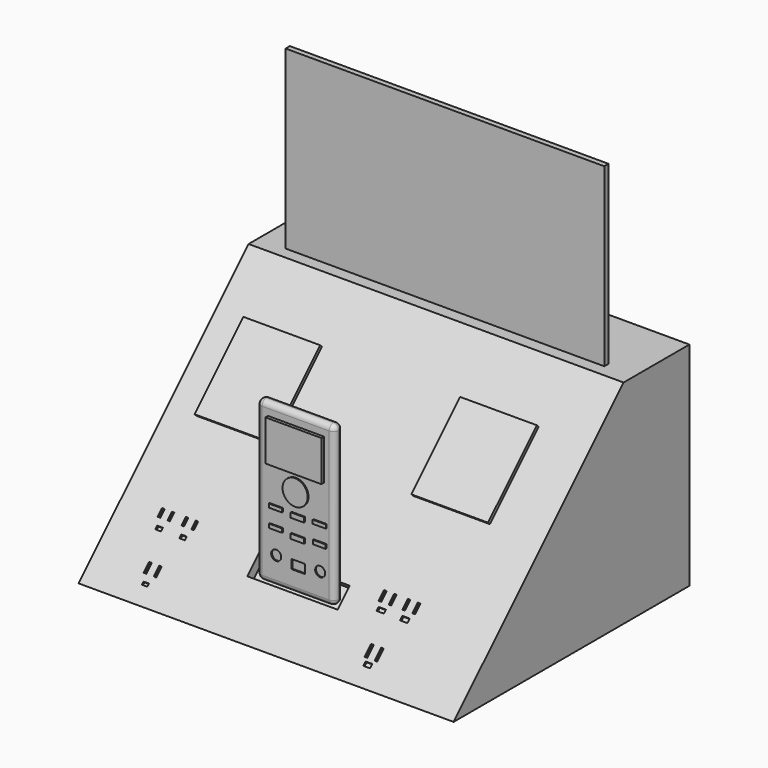
from build123d import *

# Parameters (mm, degrees)
F0_W        = 89.6722897887
F0_H        = 83.1693373621
F1_DEPTH    = 50.8
F2_T1_DEPTH = 416.2760292604
F3_W        = 76.2
F3_H        = 43.1307795863
F3_W_2      = 71.1710825562
F3_H_2      = 38.9251615852
F4_DEPTH    = 1.27
F6_W        = 18.5573295755
F6_H        = 38.1
F7_DEPTH    = 2.54
F8_R        = 1.26999
F9_W        = 21.59
F9_H        = 5.08
F10_DEPTH   = 2.286
F12_W       = 13.3995525539
F12_H       = 9.7150541842
F13_DEPTH   = 0.762
F14_R       = 3.0038864934
F14_W       = 3.1496
F14_H       = 0.8712593356
F14_W_2     = 3.1582112424
F14_H_2     = 1.159792766
F14_H_3     = 0.9281598032
F14_H_4     = 1.1401046067
F14_W_3     = 3.0329849105
F15_DEPTH   = 0.254
F14_R_2     = 1.1970137193
F14_R_3     = 1.1904625541
F14_W_4     = 3.1905571232
F14_H_5     = 2.1484075114
F16_DEPTH   = 0.254
F17_W       = 18.3596722782
F17_H       = 20.6194743514
F17_W_2     = 18.347190693
F18_DEPTH   = 0.762
F19_W       = 0.6338953972
F19_H       = 1.8462874286
F19_W_2     = 1.36038661
F19_H_2     = 0.8056527004
F19_W_3     = 0.5638897419
F19_W_4     = 0.635
F19_W_5     = 1.312000677
F19_W_6     = 0.6341952831
F19_H_3     = 2.3153796792
F19_W_7     = 1.3574287295
F19_H_4     = 0.6835795939
F19_W_8     = 1.7638131976
F19_H_5     = 0.8543668082
F19_W_9     = 1.7465222627
F19_H_6     = 0.9718833026
F19_W_10    = 1.6376990825
F19_H_7     = 0.9474921972
F19_H_8     = 2.7640033513
F19_H_9     = 2.2806219058
F20_DEPTH   = 0.508


# Not quite as in the source:
# - a fillet or chamfer that OpenCascade refuses, or shapes differently, is made with other operations: its cross-section is extruded or revolved along the edge and cut away or added
# - a fillet or chamfer is up to 0.001 mm smaller than in the source, because OpenCascade refuses the exact size
# - a feature names something its author has since deleted; it is built from what else it names


with BuildPart() as f1:
    # F0 (on Top) → F1 (new body)
    with BuildSketch(Plane.XY):
        with Locations((-0.0743344426, 4.1711423546)):
            Rectangle(F0_W, F0_H)
    extrude(amount=F1_DEPTH)

    # F2: chamfer of 63.5 on 1 edges, made by hand

    # F2_s2 → F2_t1 (cut)
    with BuildSketch(Plane.YZ.offset(-208.2123490728)):
        Polygon((-37.4135263264, -12.7), (26.0864736736, 50.8), (-37.4135263264, 50.8), align=None)
    extrude(amount=F2_T1_DEPTH, mode=Mode.SUBTRACT)

    # F9 (on face) → F10 (cut)
    with BuildSketch(Plane(origin=(0, -12.3567631632, 12.3567631632), x_dir=(1, 0, 0), z_dir=(0, -0.7071067812, 0.7071067812))):
        with Locations((-0.7835186426, -2.54)):
            Rectangle(F9_W, F9_H)
    extrude(amount=-F10_DEPTH, mode=Mode.SUBTRACT)

    # F17 (on face) → F18 (join)
    with BuildSketch(Plane(origin=(0, -12.3567631632, 12.3567631632), x_dir=(1, 0, 0), z_dir=(0, -0.7071067812, 0.7071067812))):
        with Locations((-28.8934614509, 30.5461250246)):
            Rectangle(F17_W, F17_H)
        with Locations((22.915023379, 30.5461250246)):
            Rectangle(F17_W_2, F17_H)
    extrude(amount=F18_DEPTH)

    # F19 (on face) → F20 (cut)
    with BuildSketch(Plane(origin=(0, -12.3567631632, 12.3567631632), x_dir=(1, 0, 0), z_dir=(0, -0.7071067812, 0.7071067812))):
        with Locations((-35.3719479251, 0.5594579125)):
            Rectangle(F19_W, F19_H)
        with Locations((-34.2016369104, -2.3646245245)):
            Rectangle(F19_W_2, F19_H_2)
        with Locations((-33.0321675944, 0.5594579125)):
            Rectangle(F19_W_3, F19_H)
        with Locations((-29.7049513409, 0.5594579125)):
            Rectangle(F19_W_4, F19_H)
        with Locations((-28.4958267584, -2.3646245245)):
            Rectangle(F19_W_5, F19_H_2)
        with Locations((-27.3177536994, 0.5594579125)):
            Rectangle(F19_W_6, F19_H)
        with Locations((-32.5370513409, -10.1377721876)):
            Rectangle(F19_W_4, F19_H_3)
        with Locations((-30.1494513409, -10.1377721876)):
            Rectangle(F19_W_4, F19_H_3)
        with Locations((-31.3502401114, -13.1960129365)):
            Rectangle(F19_W_7, F19_H_4)
        with Locations((18.856195733, -2.3010592558)):
            Rectangle(F19_W_8, F19_H_5)
        with Locations((24.5700171217, -2.3900355445)):
            Rectangle(F19_W_9, F19_H_6)
        with Locations((21.6742744669, -12.9482550547)):
            Rectangle(F19_W_10, F19_H_7)
        with Locations((20.5547505667, -10.3620840237)):
            Rectangle(F19_W_4, F19_H_8)
        with Locations((23.3868505667, 0.3422906739)):
            Rectangle(F19_W_4, F19_H_9)
        with Locations((25.7744505667, 0.3422906739)):
            Rectangle(F19_W_4, F19_H_9)
        with Locations((20.1102505667, 0.3422906739)):
            Rectangle(F19_W_4, F19_H_9)
        with Locations((17.7226505667, 0.3422906739)):
            Rectangle(F19_W_4, F19_H_9)
        with Locations((22.9423505667, -10.3620840237)):
            Rectangle(F19_W_4, F19_H_8)
    extrude(amount=-F20_DEPTH, mode=Mode.SUBTRACT)


with BuildPart() as f4:
    # F3 (on Front) → F4 (new body)
    with BuildSketch(Plane.XZ):
        with Locations((155.4523706436, 11.9087519124)):
            Rectangle(F3_W, F3_H)
        with Locations((155.8867506683, 11.7788566276)):
            Rectangle(F3_W_2, F3_H_2, mode=Mode.SUBTRACT)
        with Locations((155.8867506683, 11.7788566276)):
            Rectangle(F3_W_2, F3_H_2)
    extrude(amount=F4_DEPTH)


with BuildPart() as f4_1:
    # F5: moved
    add(f4.part.moved(Location((-155.702, 30.226, 59.436))))


with BuildPart() as f7:
    # F6 (on Front) → F7 (new body)
    with BuildSketch(Plane.XZ):
        with Locations((84.5490321517, 24.8106517829)):
            Rectangle(F6_W, F6_H)
    extrude(amount=F7_DEPTH)

    # F8 (radius 1.27 in the source; OpenCascade refuses exactly that, so slightly less here)
    f8_edges = [f7.edges().sort_by_distance(p)[0] for p in [
        (75.270367, 0, 24.810652),
        (75.270367, -2.54, 24.810652),
        (93.827697, 0, 24.810652),
        (93.827697, -2.54, 24.810652),
        (75.270367, -1.27, 5.760652),
        (93.827697, -1.27, 5.760652),
        (84.549032, 0, 5.760652),
        (84.549032, -2.54, 5.760652),
        (93.827697, -1.27, 43.860652),
        (75.270367, -1.27, 43.860652),
        (84.549032, 0, 43.860652),
        (84.549032, -2.54, 43.860652),
    ]]
    fillet(f8_edges, radius=F8_R)


with BuildPart() as f7_1:
    # F11: moved
    add(f7.part.moved(Location((-85.344, -12.446, 2.4892))))

    # F12 (on face) → F13 (join)
    with BuildSketch(Plane.XZ.offset(14.986)):
        with Locations((-0.7233838551, 38.6430229992)):
            Rectangle(F12_W, F12_H)
    extrude(amount=F13_DEPTH)

    # F14 (on face) → F15 (join)
    with BuildSketch(Plane.XZ.offset(14.986)):
        with Locations((-0.7233838551, 29.6452492476)):
            Circle(F14_R)
        with Locations((-5.446629824, 24.857554393)):
            Rectangle(F14_W, F14_H)
        with Locations((-0.1904759556, 24.5668822899)):
            Rectangle(F14_W_2, F14_H_2)
        with Locations((5.0665399105, 24.857554393)):
            Rectangle(F14_W, F14_H)
        with Locations((-5.446629824, 20.6073820591)):
            Rectangle(F14_W, F14_H_3)
        with Locations((-0.1904759556, 20.1132884249)):
            Rectangle(F14_W_2, F14_H_4)
        with Locations((5.062614684, 20.6073820591)):
            Rectangle(F14_W_3, F14_H_3)
    extrude(amount=F15_DEPTH)

    # F14 (on face) → F16 (cut)
    with BuildSketch(Plane.XZ.offset(14.986)):
        with Locations((-5.446629824, 14.7840231657)):
            Circle(F14_R_2)
        with Locations((5.062614684, 14.7840231657)):
            Circle(F14_R_3)
        with Locations((-0.1743030152, 14.144777786)):
            Rectangle(F14_W_4, F14_H_5)
    extrude(amount=-F16_DEPTH, mode=Mode.SUBTRACT)


solid = Compound([f1.part, f4_1.part, f7_1.part])
